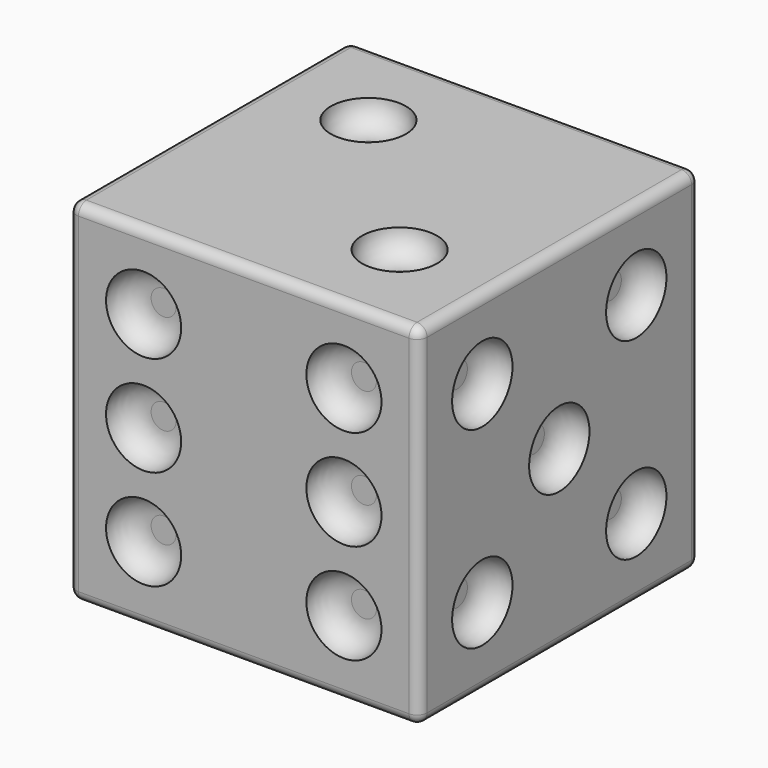
from build123d import *

# Parameters (mm, degrees)
F0_R      = 127
F1_DEPTH  = 177.8
F2_R      = 127
F2_W      = 177.8
F2_H      = 177.8
F3_DEPTH  = 177.801
F4_R      = 19.1220202056
F5_DEPTH  = 12.7
F6_R      = 19.05
F7_DEPTH  = 12.7
F8_R      = 19.05
F9_DEPTH  = 12.7
F10_R     = 19.05
F11_DEPTH = 12.7
F12_R     = 19.05
F13_DEPTH = 12.7
F14_R     = 19.05
F15_DEPTH = 12.7
F16_R     = 12.69999
F17_R     = 5.08


# Not quite as in the source:
# - a fillet or chamfer is up to 0.001 mm smaller than in the source, because OpenCascade refuses the exact size
# - a pattern or mirror of a feature is missing from the dataset's text; its kind, count and spacing are read off the source's solid
# - a feature names something its author has since deleted; it is built from what else it names


with BuildPart() as f1:
    # F0 (on Top) → F1 (new body)
    with BuildSketch(Plane.XY):
        Circle(F0_R)
    extrude(amount=F1_DEPTH)

    # F2 (on face) → F3 (cut, through all)
    with BuildSketch(Plane.XY.offset(177.8)):
        Circle(F2_R)
        Rectangle(F2_W, F2_H, mode=Mode.SUBTRACT)
    extrude(amount=-F3_DEPTH, mode=Mode.SUBTRACT)

    # F4 (on face) → F5 (cut)
    with BuildSketch(Plane.YZ.offset(88.9)):
        with Locations((-48.7996374987, 137.6996374987)):
            Circle(F4_R)
        with Locations((0, 88.9)):
            Circle(F4_R)
        with Locations((48.7996374987, 137.6996374987)):
            Circle(F4_R)
        with Locations((48.7996374987, 40.1003625013)):
            Circle(F4_R)
        with Locations((-48.7996374987, 40.1003625013)):
            Circle(F4_R)
    extrude(amount=-F5_DEPTH, mode=Mode.SUBTRACT)

    # F6 (on face) → F7 (cut)
    with BuildSketch(Plane.XZ.offset(88.9)):
        with Locations((-50.8, 88.9)):
            Circle(F6_R)
        with Locations((50.8, 88.9)):
            Circle(F6_R)
    f7 = extrude(amount=-F7_DEPTH, mode=Mode.SUBTRACT)

    # F7_copies: F7 across plane
    add(f7.mirror(Plane.XY.offset(114.3)), mode=Mode.SUBTRACT)

    # F7_copies1: F7 across plane
    add(f7.mirror(Plane(origin=(0, 0, 63.5), x_dir=(-1, 0, 0), z_dir=(0, 0, -1))), mode=Mode.SUBTRACT)

    # F8 (on face) → F9 (cut)
    with BuildSketch(Plane(origin=(-88.9, 0, 0), x_dir=(0, -1, 0), z_dir=(-1, 0, 0))):
        with Locations((50.8, 38.1)):
            Circle(F8_R)
        with Locations((-50.8, 38.1)):
            Circle(F8_R)
        with Locations((-50.8, 139.7)):
            Circle(F8_R)
        with Locations((50.8, 139.7)):
            Circle(F8_R)
    extrude(amount=-F9_DEPTH, mode=Mode.SUBTRACT)

    # F10 (on face) → F11 (cut)
    with BuildSketch(Plane(origin=(0, 88.9, 0), x_dir=(-1, 0, 0), z_dir=(0, 1, 0))):
        with Locations((50.8, 38.1)):
            Circle(F10_R)
        with Locations((0, 88.9)):
            Circle(F10_R)
        with Locations((-50.8, 139.7)):
            Circle(F10_R)
    extrude(amount=-F11_DEPTH, mode=Mode.SUBTRACT)

    # F12 (on face) → F13 (cut)
    with BuildSketch(Plane(origin=(0, 0, 0), x_dir=(1, 0, 0), z_dir=(0, 0, -1))):
        Circle(F12_R)
    extrude(amount=-F13_DEPTH, mode=Mode.SUBTRACT)

    # F14 (on face) → F15 (cut)
    with BuildSketch(Plane.XY.offset(177.8)):
        with Locations((-39.5085913341, 39.5085913341)):
            Circle(F14_R)
        with Locations((39.5085913341, -39.5085913341)):
            Circle(F14_R)
    extrude(amount=-F15_DEPTH, mode=Mode.SUBTRACT)

    # F16 (radius 12.7 in the source; OpenCascade refuses exactly that, so slightly less here)
    f16_edges = [f1.edges().sort_by_distance(p)[0] for p in [
        (76.2, -67.921658, 137.699637),
        (76.2, -19.12202, 88.9),
        (76.2, 29.677617, 137.699637),
        (76.2, -67.921658, 40.100363),
        (76.2, 29.677617, 40.100363),
        (31.75, -76.2, 38.1),
        (-69.85, -76.2, 38.1),
        (31.75, -76.2, 88.9),
        (31.75, -76.2, 139.7),
        (-69.85, -76.2, 88.9),
        (-69.85, -76.2, 139.7),
        (-76.2, -31.75, 38.1),
        (-76.2, 69.85, 38.1),
        (-76.2, 69.85, 139.7),
        (-76.2, -31.75, 139.7),
        (19.05, 76.2, 88.9),
        (69.85, 76.2, 139.7),
        (-31.75, 76.2, 38.1),
        (-19.05, 0, 12.7),
        (-58.558591, 39.508591, 165.1),
        (20.458591, -39.508591, 165.1),
    ]]
    fillet(f16_edges, radius=F16_R)

    # F17
    f17_edges = [f1.edges().sort_by_distance(p)[0] for p in [
        (0, -88.9, 177.8),
        (88.9, 0, 177.8),
        (88.9, -88.9, 88.9),
        (0, 88.9, 177.8),
        (-88.9, 0, 177.8),
        (-88.9, -88.9, 88.9),
        (-88.9, 88.9, 88.9),
        (-88.9, 0, 0),
        (0, -88.9, 0),
        (88.9, 0, 0),
        (0, 88.9, 0),
        (88.9, 88.9, 88.9),
    ]]
    fillet(f17_edges, radius=F17_R)


solid = f1.part
